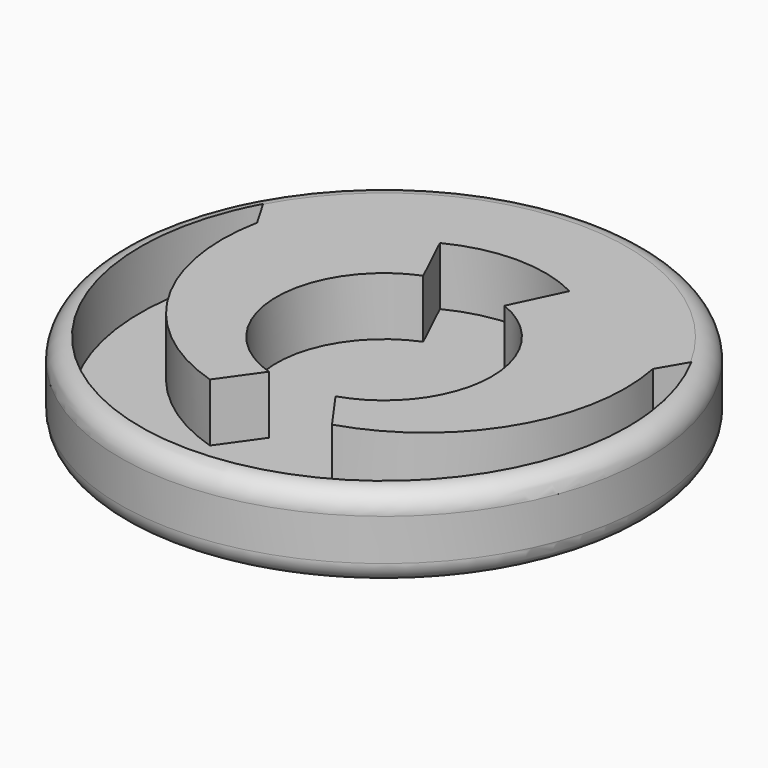
from build123d import *

# Parameters (mm, degrees)
F0_R     = 80.6856028543
F1_DEPTH = 25.4
F2_DEPTH = 7.62


# Not quite as in the source:
# - a fillet or chamfer that OpenCascade refuses, or shapes differently, is made with other operations: its cross-section is extruded or revolved along the edge and cut away or added


with BuildPart() as f1:
    # F0 (on Top) → F1 (new body)
    with BuildSketch(Plane.XY):
        Circle(F0_R)
        with BuildLine():
            ThreePointArc((65.4481636504, 35.6006994652), (72.2046857665, 18.3672338959), (74.5041738939, 0))
            ThreePointArc((74.5041738939, 0), (-18.3672338959, -72.2046857665), (-65.4481636504, 35.6006994652))
            ThreePointArc((-65.4481636504, 35.6006994652), (0, 74.5041738939), (65.4481636504, 35.6006994652))
        make_face(mode=Mode.SUBTRACT)
        with BuildLine():
            Line((60.4875776026, 27.0912961706), (65.4481636504, 35.6006994652))
            ThreePointArc((65.4481636504, 35.6006994652), (0, 74.5041738939), (-65.4481636504, 35.6006994652))
            Line((-65.4481636504, 35.6006994652), (-60.4875776026, 27.0912961706))
            ThreePointArc((-60.4875776026, 27.0912961706), (-53.0522524477, -16.0833720047), (-18.6689998955, -43.2334728539))
            Line((-18.6689998955, -43.2334728539), (-10.1934868934, -31.2953587769))
            ThreePointArc((-10.1934868934, -31.2953587769), (-32.8922648635, -1.1855666041), (-12.4201237339, 30.4802753015))
            Line((-12.4201237339, 30.4802753015), (-19.8746794874, 46.1712545885))
            ThreePointArc((-19.8746794874, 46.1712545885), (-0.0120295356, 50.8915609087), (19.8259803172, 46.0687484571))
            Line((19.8259803172, 46.0687484571), (12.4201237339, 30.4802753015))
            ThreePointArc((12.4201237339, 30.4802753015), (27.3138970192, 18.3645769254), (32.9136241703, 0))
            ThreePointArc((32.9136241703, 0), (26.6346696302, -19.3365206207), (10.1934868934, -31.2953587769))
            Line((10.1934868934, -31.2953587769), (18.6689998955, -43.2334728539))
            ThreePointArc((18.6689998955, -43.2334728539), (53.0522524477, -16.0833720047), (60.4875776026, 27.0912961706))
        make_face()
    extrude(amount=F1_DEPTH)

    # F0 (on Top) → F2 (join)
    with BuildSketch(Plane.XY):
        with BuildLine():
            ThreePointArc((-10.1934868934, -31.2953587769), (0, -32.9136241703), (10.1934868934, -31.2953587769))
            ThreePointArc((10.1934868934, -31.2953587769), (26.6346696302, -19.3365206207), (32.9136241703, 0))
            ThreePointArc((32.9136241703, 0), (27.3138970192, 18.3645769254), (12.4201237339, 30.4802753015))
            ThreePointArc((12.4201237339, 30.4802753015), (0, 32.9136241703), (-12.4201237339, 30.4802753015))
            ThreePointArc((-12.4201237339, 30.4802753015), (-32.8922648635, -1.1855666041), (-10.1934868934, -31.2953587769))
        make_face()
        with BuildLine():
            Line((-19.8746794874, 46.1712545885), (-12.4201237339, 30.4802753015))
            ThreePointArc((-12.4201237339, 30.4802753015), (0, 32.9136241703), (12.4201237339, 30.4802753015))
            Line((12.4201237339, 30.4802753015), (19.8259803172, 46.0687484571))
            ThreePointArc((19.8259803172, 46.0687484571), (-0.0120295356, 50.8915609087), (-19.8746794874, 46.1712545885))
        make_face()
        with BuildLine():
            ThreePointArc((-65.4481636504, 35.6006994652), (-18.3672338959, -72.2046857665), (74.5041738939, 0))
            ThreePointArc((74.5041738939, 0), (72.2046857665, 18.3672338959), (65.4481636504, 35.6006994652))
            Line((65.4481636504, 35.6006994652), (60.4875776026, 27.0912961706))
            ThreePointArc((60.4875776026, 27.0912961706), (53.0522524477, -16.0833720047), (18.6689998955, -43.2334728539))
            Line((18.6689998955, -43.2334728539), (10.1934868934, -31.2953587769))
            ThreePointArc((10.1934868934, -31.2953587769), (0, -32.9136241703), (-10.1934868934, -31.2953587769))
            Line((-10.1934868934, -31.2953587769), (-18.6689998955, -43.2334728539))
            ThreePointArc((-18.6689998955, -43.2334728539), (-53.0522524477, -16.0833720047), (-60.4875776026, 27.0912961706))
            Line((-60.4875776026, 27.0912961706), (-65.4481636504, 35.6006994652))
        make_face()
    extrude(amount=F2_DEPTH)

    # F3: fillet of radius 6.35 on 2 edges, made by hand

    # F3_s1 → F3_t2 (revolve, cut)
    with BuildSketch(Plane.XZ):
        with BuildLine():
            ThreePointArc((80.6856028543, 19.05), (78.8257309148, 23.5401280605), (74.3356028543, 25.4))
            Line((74.3356028543, 25.4), (74.3356028543, 25.527))
            Line((74.3356028543, 25.527), (80.8126028543, 25.527))
            Line((80.8126028543, 25.527), (80.8126028543, 19.05))
            Line((80.8126028543, 19.05), (80.6856028543, 19.05))
        make_face()
    revolve(axis=Axis((0, 0, 25.4), (0, 0, 1)), mode=Mode.SUBTRACT)

    # F3_s3 → F3_t4 (revolve, cut)
    with BuildSketch(Plane.XZ):
        with BuildLine():
            ThreePointArc((80.6856028543, 6.35), (78.8257309148, 1.8598719395), (74.3356028543, 0))
            Line((74.3356028543, 0), (74.3356028543, -0.127))
            Line((74.3356028543, -0.127), (80.8126028543, -0.127))
            Line((80.8126028543, -0.127), (80.8126028543, 6.35))
            Line((80.8126028543, 6.35), (80.6856028543, 6.35))
        make_face()
    revolve(axis=Axis((0, 0, 0), (0, 0, 1)), mode=Mode.SUBTRACT)


solid = f1.part
